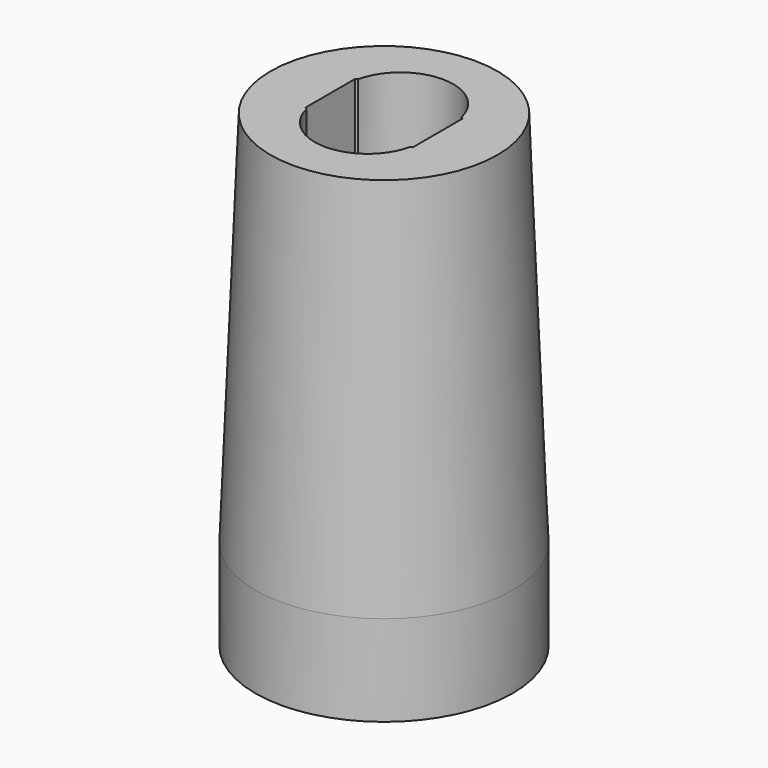
from build123d import *

# Parameters (mm, degrees)
F0_R         = 8.5
F1_DEPTH     = 16
F2_DEPTH     = 4
F3_DEPTH     = 15
F4_W         = 9.6
F4_H         = 9.6
F5_DEPTH     = 11
F6_T1_DEPTH  = 10
F6_T3_DEPTH  = 7.6
F6_T5_DEPTH  = 7.6
F6_S9_W      = 1.02
F6_S9_H      = 1.02
F6_T10_DEPTH = 1.02
F6_S15_W     = 1.02
F6_S15_H     = 1.02
F6_T16_DEPTH = 1.02
F6_S21_W     = 1.02
F6_S21_H     = 1.02
F6_T22_DEPTH = 1.02
F6_S27_W     = 1.02
F6_S27_H     = 1.02
F6_T28_DEPTH = 1.02
F7_SIZE2     = 25
F7_SIZE      = 1
F8_T1_DEPTH  = 4
F8_T3_DEPTH  = 4
F9_DEPTH     = 25


# Not quite as in the source:
# - a fillet or chamfer that OpenCascade refuses, or shapes differently, is made with other operations: its cross-section is extruded or revolved along the edge and cut away or added


with BuildPart() as f1:
    # F0 (on Top) → F1 (new body)
    with BuildSketch(Plane.XY):
        Circle(F0_R)
        with BuildLine():
            Line((3.4119543857, 2.130107217), (3.5507041555, 2.05))
            Line((3.5507041555, 2.05), (3.5507041555, -2.05))
            Line((3.5507041555, -2.05), (3.4119543857, -2.130107217))
            ThreePointArc((3.4119543857, -2.130107217), (0, -4.85), (-3.4119543857, -2.130107217))
            Line((-3.4119543857, -2.130107217), (-3.5507041555, -2.05))
            Line((-3.5507041555, -2.05), (-3.5507041555, 2.05))
            Line((-3.5507041555, 2.05), (-3.4119543857, 2.130107217))
            ThreePointArc((-3.4119543857, 2.130107217), (0, 4.85), (3.4119543857, 2.130107217))
        make_face(mode=Mode.SUBTRACT)
    extrude(amount=F1_DEPTH)

    # F0 (on Top) → F2 (join)
    with BuildSketch(Plane.XY):
        with BuildLine():
            Line((0, 4.1), (3.4119543857, 2.130107217))
            ThreePointArc((3.4119543857, 2.130107217), (0, 4.85), (-3.4119543857, 2.130107217))
            Line((-3.4119543857, 2.130107217), (0, 4.1))
        make_face()
        with BuildLine():
            ThreePointArc((-3.4119543857, -2.130107217), (0, -4.85), (3.4119543857, -2.130107217))
            Line((3.4119543857, -2.130107217), (0, -4.1))
            Line((0, -4.1), (-3.4119543857, -2.130107217))
        make_face()
    extrude(amount=F2_DEPTH)

    # F0 (on Top) → F3 (join)
    with BuildSketch(Plane.XY):
        Circle(F0_R)
        with BuildLine():
            Line((3.4119543857, 2.130107217), (3.5507041555, 2.05))
            Line((3.5507041555, 2.05), (3.5507041555, -2.05))
            Line((3.5507041555, -2.05), (3.4119543857, -2.130107217))
            ThreePointArc((3.4119543857, -2.130107217), (0, -4.85), (-3.4119543857, -2.130107217))
            Line((-3.4119543857, -2.130107217), (-3.5507041555, -2.05))
            Line((-3.5507041555, -2.05), (-3.5507041555, 2.05))
            Line((-3.5507041555, 2.05), (-3.4119543857, 2.130107217))
            ThreePointArc((-3.4119543857, 2.130107217), (0, 4.85), (3.4119543857, 2.130107217))
        make_face(mode=Mode.SUBTRACT)
        with BuildLine():
            ThreePointArc((-3.5, 1.35), (-3.4779189431, 1.7425300307), (-3.4119543857, 2.130107217))
            Line((-3.4119543857, 2.130107217), (-3.5507041555, 2.05))
            Line((-3.5507041555, 2.05), (-3.5507041555, -2.05))
            Line((-3.5507041555, -2.05), (-3.4119543857, -2.130107217))
            ThreePointArc((-3.4119543857, -2.130107217), (-3.4779189431, -1.7425300307), (-3.5, -1.35))
            Line((-3.5, -1.35), (-3.5, 1.35))
        make_face()
        with BuildLine():
            Line((0, 4.1), (3.4119543857, 2.130107217))
            ThreePointArc((3.4119543857, 2.130107217), (0, 4.85), (-3.4119543857, 2.130107217))
            Line((-3.4119543857, 2.130107217), (0, 4.1))
        make_face()
        with BuildLine():
            ThreePointArc((-3.4119543857, -2.130107217), (0, -4.85), (3.4119543857, -2.130107217))
            Line((3.4119543857, -2.130107217), (0, -4.1))
            Line((0, -4.1), (-3.4119543857, -2.130107217))
        make_face()
        with BuildLine():
            Line((3.5507041555, -2.05), (3.5507041555, 2.05))
            Line((3.5507041555, 2.05), (3.4119543857, 2.130107217))
            ThreePointArc((3.4119543857, 2.130107217), (3.4779189431, 1.7425300307), (3.5, 1.35))
            Line((3.5, 1.35), (3.5, -1.35))
            ThreePointArc((3.5, -1.35), (3.4779189431, -1.7425300307), (3.4119543857, -2.130107217))
            Line((3.4119543857, -2.130107217), (3.5507041555, -2.05))
        make_face()
    extrude(amount=-F3_DEPTH)

    # F4 (on face) → F5 (cut)
    with BuildSketch(Plane(origin=(0, 0, -15), x_dir=(1, 0, 0), z_dir=(0, 0, -1))):
        Rectangle(F4_W, F4_H)
        with BuildLine():
            Line((-3.4119543857, 2.130107217), (0, 4.1))
            Line((0, 4.1), (3.4119543857, 2.130107217))
            ThreePointArc((3.4119543857, 2.130107217), (3.4779189431, 1.7425300307), (3.5, 1.35))
            Line((3.5, 1.35), (3.5, -1.35))
            ThreePointArc((3.5, -1.35), (3.4779189431, -1.7425300307), (3.4119543857, -2.130107217))
            Line((3.4119543857, -2.130107217), (0, -4.1))
            Line((0, -4.1), (-3.4119543857, -2.130107217))
            ThreePointArc((-3.4119543857, -2.130107217), (-3.4779189431, -1.7425300307), (-3.5, -1.35))
            Line((-3.5, -1.35), (-3.5, 1.35))
            ThreePointArc((-3.5, 1.35), (-3.4779189431, 1.7425300307), (-3.4119543857, 2.130107217))
        make_face(mode=Mode.SUBTRACT)
    extrude(amount=-F5_DEPTH, mode=Mode.SUBTRACT)

    # F6: fillet of radius 1 on 8 edges, made by hand

    # F6_s2 → F6_t1 (join)
    with BuildSketch(Plane.XY.offset(-15)):
        with BuildLine():
            ThreePointArc((-4.8, -3.8), (-4.5071067812, -4.5071067812), (-3.8, -4.8))
            Line((-3.8, -4.8), (-4.8, -4.8))
            Line((-4.8, -4.8), (-4.8, -3.8))
        make_face()
        with BuildLine():
            ThreePointArc((-4.8, 3.8), (-4.5071067812, 4.5071067812), (-3.8, 4.8))
            Line((-3.8, 4.8), (-4.8, 4.8))
            Line((-4.8, 4.8), (-4.8, 3.8))
        make_face()
        with BuildLine():
            ThreePointArc((3.8, -4.8), (4.5071067812, -4.5071067812), (4.8, -3.8))
            Line((4.8, -3.8), (4.8, -4.8))
            Line((4.8, -4.8), (3.8, -4.8))
        make_face()
        with BuildLine():
            ThreePointArc((4.8, 3.8), (4.5071067812, 4.5071067812), (3.8, 4.8))
            Line((3.8, 4.8), (4.8, 4.8))
            Line((4.8, 4.8), (4.8, 3.8))
        make_face()
    extrude(amount=F6_T1_DEPTH)

    # F6_s4 → F6_t3 (join)
    with BuildSketch(Plane.YZ.offset(-3.8)):
        with BuildLine():
            ThreePointArc((4.8, -5), (4.5071067812, -4.2928932188), (3.8, -4))
            Line((3.8, -4), (4.8, -4))
            Line((4.8, -4), (4.8, -5))
        make_face()
        with BuildLine():
            ThreePointArc((-4.8, -5), (-4.5071067812, -4.2928932188), (-3.8, -4))
            Line((-3.8, -4), (-4.8, -4))
            Line((-4.8, -4), (-4.8, -5))
        make_face()
    extrude(amount=F6_T3_DEPTH)

    # F6_s6 → F6_t5 (join)
    with BuildSketch(Plane.XZ.offset(-3.8)):
        with BuildLine():
            ThreePointArc((-4.8, -5), (-4.5071067812, -4.2928932188), (-3.8, -4))
            Line((-3.8, -4), (-4.8, -4))
            Line((-4.8, -4), (-4.8, -5))
        make_face()
        with BuildLine():
            ThreePointArc((4.8, -5), (4.5071067812, -4.2928932188), (3.8, -4))
            Line((3.8, -4), (4.8, -4))
            Line((4.8, -4), (4.8, -5))
        make_face()
    extrude(amount=F6_T5_DEPTH)


with BuildPart() as f6_tool8:
    # F6_s9 → F6_t10 (new body)
    with BuildSketch(Plane.XY.offset(-5)):
        with Locations((-4.31, -4.31)):
            Rectangle(F6_S9_W, F6_S9_H)
    extrude(amount=F6_T10_DEPTH)

    # F6_s11 → F6_t12 (revolve, cut)
    with BuildSketch(Plane(origin=(-3.8, -3.8, -5), x_dir=(0.7071067812, 0.7071067812, 0), z_dir=(0.7071067812, -0.7071067812, 0))):
        with BuildLine():
            ThreePointArc((0, -1), (1, 0), (0, 1))
            Line((0, 1), (0, -1))
        make_face()
    revolve(axis=Axis((-3.8, -3.8, -5), (0, 0, 1)), mode=Mode.SUBTRACT)


with BuildPart() as f1_1:
    add(f1.part)

    # F6_t7: union F6_tool8
    add(f6_tool8.part)


with BuildPart() as f6_tool14:
    # F6_s15 → F6_t16 (new body)
    with BuildSketch(Plane.XY.offset(-5)):
        with Locations((-4.31, 4.31)):
            Rectangle(F6_S15_W, F6_S15_H)
    extrude(amount=F6_T16_DEPTH)

    # F6_s17 → F6_t18 (revolve, cut)
    with BuildSketch(Plane(origin=(-3.8, 3.8, -5), x_dir=(0.7071067812, -0.7071067812, 0), z_dir=(-0.7071067812, -0.7071067812, 0))):
        with BuildLine():
            ThreePointArc((0, -1), (1, 0), (0, 1))
            Line((0, 1), (0, -1))
        make_face()
    revolve(axis=Axis((-3.8, 3.8, -5), (0, 0, 1)), mode=Mode.SUBTRACT)


with BuildPart() as f1_2:
    add(f1_1.part)

    # F6_t13: union F6_tool14
    add(f6_tool14.part)


with BuildPart() as f6_tool20:
    # F6_s21 → F6_t22 (new body)
    with BuildSketch(Plane.XY.offset(-5)):
        with Locations((4.31, -4.31)):
            Rectangle(F6_S21_W, F6_S21_H)
    extrude(amount=F6_T22_DEPTH)

    # F6_s23 → F6_t24 (revolve, cut)
    with BuildSketch(Plane(origin=(3.8, -3.8, -5), x_dir=(-0.7071067812, 0.7071067812, 0), z_dir=(0.7071067812, 0.7071067812, 0))):
        with BuildLine():
            ThreePointArc((0, -1), (1, 0), (0, 1))
            Line((0, 1), (0, -1))
        make_face()
    revolve(axis=Axis((3.8, -3.8, -5), (0, 0, 1)), mode=Mode.SUBTRACT)


with BuildPart() as f1_3:
    add(f1_2.part)

    # F6_t19: union F6_tool20
    add(f6_tool20.part)


with BuildPart() as f6_tool26:
    # F6_s27 → F6_t28 (new body)
    with BuildSketch(Plane.XY.offset(-5)):
        with Locations((4.31, 4.31)):
            Rectangle(F6_S27_W, F6_S27_H)
    extrude(amount=F6_T28_DEPTH)

    # F6_s29 → F6_t30 (revolve, cut)
    with BuildSketch(Plane(origin=(3.8, 3.8, -5), x_dir=(-0.7071067812, -0.7071067812, 0), z_dir=(-0.7071067812, 0.7071067812, 0))):
        with BuildLine():
            ThreePointArc((0, -1), (1, 0), (0, 1))
            Line((0, 1), (0, -1))
        make_face()
    revolve(axis=Axis((3.8, 3.8, -5), (0, 0, 1)), mode=Mode.SUBTRACT)


with BuildPart() as f1_4:
    add(f1_3.part)

    # F6_t25: union F6_tool26
    add(f6_tool26.part)

    # F7
    f7_edges = [f1_4.edges().sort_by_distance(p)[0] for p in [
        (-8.5, 0, 16),
    ]]
    f7_side = f1_4.faces().sort_by_distance((-8.259584, 0, 16))[0]
    chamfer(f7_edges, length=F7_SIZE, length2=F7_SIZE2, reference=f7_side)

    # F8: fillet of radius 5 on 4 edges, made by hand

    # F8_s2 → F8_t1 (join)
    with BuildSketch(Plane.XY):
        with BuildLine():
            ThreePointArc((2.5, -2.656624327), (0, -3.3264973081), (-2.5, -2.656624327))
            Line((-2.5, -2.656624327), (0, -4.1))
            Line((0, -4.1), (2.5, -2.656624327))
        make_face()
        with BuildLine():
            ThreePointArc((2.5, 2.656624327), (0, 3.3264973081), (-2.5, 2.656624327))
            Line((-2.5, 2.656624327), (0, 4.1))
            Line((0, 4.1), (2.5, 2.656624327))
        make_face()
    extrude(amount=F8_T1_DEPTH)

    # F8_s4 → F8_t3 (join)
    with BuildSketch(Plane.XY.offset(-4)):
        with BuildLine():
            ThreePointArc((2.5, -2.656624327), (0, -3.3264973081), (-2.5, -2.656624327))
            Line((-2.5, -2.656624327), (0, -4.1))
            Line((0, -4.1), (2.5, -2.656624327))
        make_face()
        with BuildLine():
            ThreePointArc((2.5, 2.656624327), (0, 3.3264973081), (-2.5, 2.656624327))
            Line((-2.5, 2.656624327), (0, 4.1))
            Line((0, 4.1), (2.5, 2.656624327))
        make_face()
    extrude(amount=F8_T3_DEPTH)

    # F9 (cut): faces of the model
    f9_faces = [f1_4.faces().sort_by_distance(p)[0] for p in [
        (3.5168739038, 0, 0),
        (-3.5168739038, 0, 0),
    ]]
    extrude(f9_faces, amount=-F9_DEPTH, mode=Mode.SUBTRACT)


solid = f1_4.part
